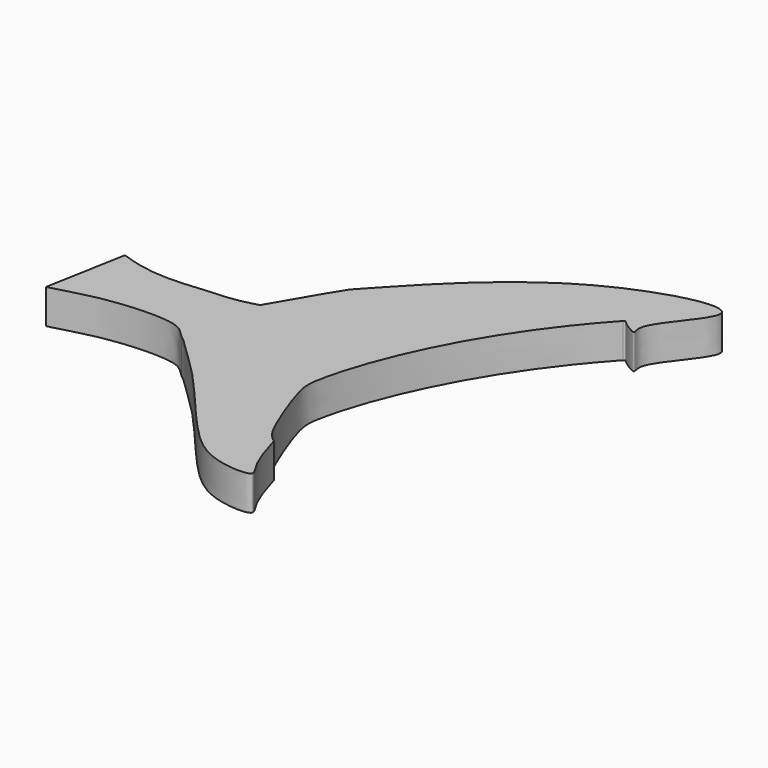
from build123d import *

# Parameters (mm, degrees)
F1_DEPTH = 25.4


with BuildPart() as f1:
    # F0 (on Top) → F1 (new body)
    with BuildSketch(Plane.XY):
        with BuildLine():
            add(Edge.make_bspline(
                [(763.0332921978, -9.3896612425), (758.8732603057, -5.7958741093), (752.748302509, 4.4572593378), (696.4067030942, 0.6728158791), (683.5044525744, -4.3029026677), (663.4436377218, -9.3896612425)],
                knots=[0, 0, 0, 0, 0.2297210344, 0.63017097, 1, 1, 1, 1], degree=3))
            add(Edge.make_bspline(
                [(763.0332921978, -9.3896612425), (766.7884226576, -11.9368133928), (779.5890477216, -25.2148041632), (800.2290337642, -43.9743335152), (839.0095670245, -91.9576915528), (867.7100367018, -118.1913476961), (906.8571338402, -119.815920499), (892.7640754987, -106.5688383093), (884.9547505379, -76.6774757721), (884.9547505379, -77.1626904607)],
                knots=[0, 0, 0, 0, 0.1179171354, 0.2600639543, 0.4629010708, 0.6319047181, 0.7652001452, 0.8594477992, 1, 1, 1, 1], degree=3))
            add(Edge.make_bspline(
                [(884.9547505379, -77.1626904607), (878.3393838169, -72.742209961), (870.6491021392, -56.1357861732), (856.2695164987, -18.1768013701), (856.1642570221, 4.1483188267), (885.188683908, 95.6630026172), (948.2003044353, 164.2756462097)],
                knots=[0, 0, 0, 0, 0.1725941963, 0.3844527192, 0.5337250947, 1, 1, 1, 1], degree=3))
            add(Edge.make_bspline(
                [(948.2003044353, 164.2756462097), (949.6786594391, 165.2318388224), (948.9464949683, 164.3876408494), (965.7476039449, 153.2811721488), (954.758612186, 167.9740501467), (1018.6311971569, 226.3796883651), (885.4114990535, 194.3808367453), (791.2197277599, 82.6677856639), (804.1064157523, 102.1605908318), (773.3094898025, 49.58736149)],
                knots=[0, 0, 0, 0, 0.032410144, 0.1167850345, 0.1807601525, 0.341583858, 0.5590195094, 0.8177158141, 1, 1, 1, 1], degree=3))
            add(Edge.make_bspline(
                [(773.3094898025, 49.58736149), (755.538612277, 44.2709080376), (735.1738345899, 46.185123763), (702.9238090782, 39.3427649071), (674.1561889648, 49.58736149)],
                knots=[0, 0, 0, 0, 0.4420458662, 1, 1, 1, 1], degree=3))
            Line((674.1561889648, 49.58736149), (663.4436377218, -9.3896612425))
        make_face()
    extrude(amount=F1_DEPTH)


solid = f1.part
